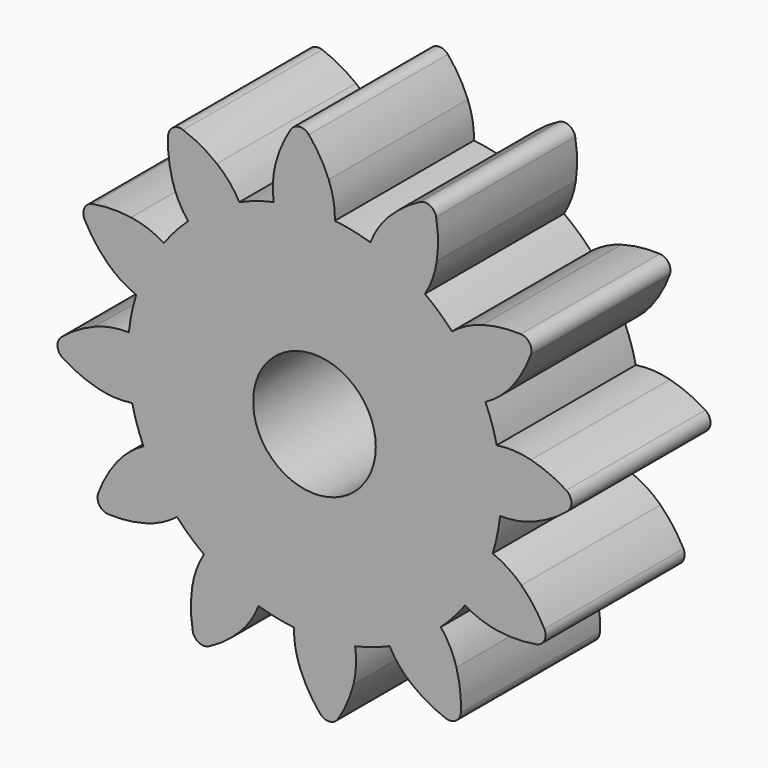
from build123d import *

# Parameters (mm, degrees)
F0_R     = 8.8190251349
F1_DEPTH = 25
F2_COUNT = 12


# Not quite as in the source:
# - a feature names something its author has since deleted; it is built from what else it names


with BuildPart() as f1:
    # F0 (on Front) → F1 (new body)
    with BuildSketch(Plane.XZ):
        with BuildLine():
            ThreePointArc((-5.8511671906, 26.2154592323), (-16.7976364993, -20.9601018196), (26.8605, 0))
            ThreePointArc((26.8605, 0), (20.0037882945, 17.9258169722), (2.9342950433, 26.6997448087))
            ThreePointArc((2.9342950433, 26.6997448087), (-1.4784007951, 26.8197835811), (-5.8511671906, 26.2154592323))
        make_face()
        Circle(F0_R, mode=Mode.SUBTRACT)
        with BuildLine():
            ThreePointArc((-5.8511671906, 26.2154592323), (-1.4784007951, 26.8197835811), (2.9342950433, 26.6997448087))
            ThreePointArc((2.9342950433, 26.6997448087), (2.7429832933, 29.2065995461), (2.0526051191, 31.6240980128))
            ThreePointArc((2.0526051191, 31.6240980128), (0.8166449435, 34.1202908544), (-0.8038354447, 36.3858193952))
            ThreePointArc((-0.8038354447, 36.3858193952), (-2.1425207788, 36.9553506751), (-3.3954147249, 36.215958315))
            ThreePointArc((-3.3954147249, 36.215958315), (-4.7063208649, 33.7582965503), (-5.6058886832, 31.122133809))
            ThreePointArc((-5.6058886832, 31.122133809), (-5.9726089783, 28.6809978257), (-5.8511671906, 26.2154592323))
        make_face()
    extrude(amount=F1_DEPTH)

    # F2: F1 ×12 about axis
    f2_axis = Axis((0, 0, 0), (0, 1, 0))


with BuildPart() as f1_1:
    add(f1.part)
    for i in range(1, F2_COUNT):
        add(f1.part.rotate(f2_axis, i * 360 / F2_COUNT))


solid = f1_1.part
